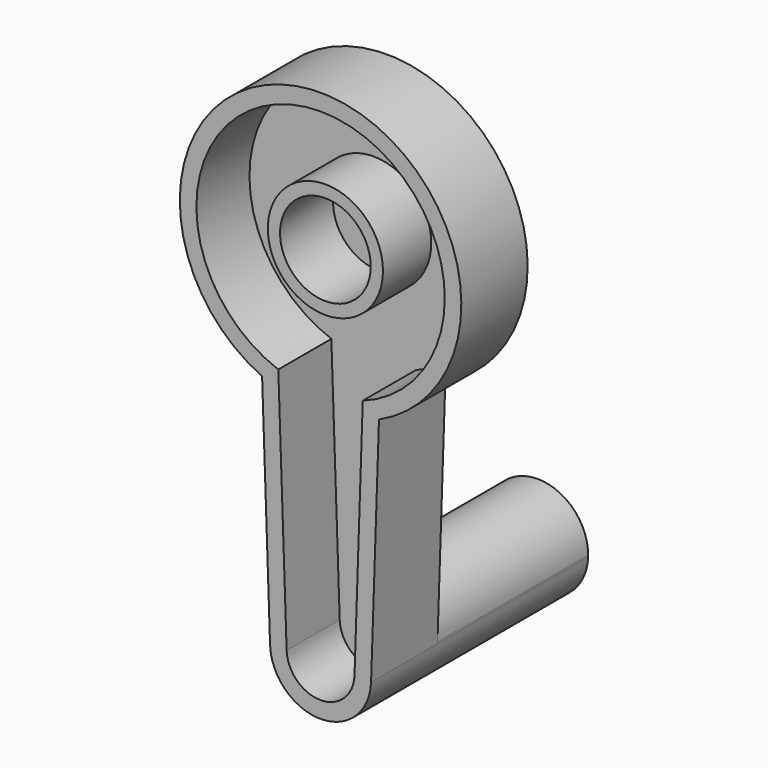
from build123d import *

# Parameters (mm, degrees)
F0_R     = 5.0192291216
F1_DEPTH = 11
F2_T     = -2.2
F3_R     = 7.6408252188
F4_DEPTH = 8
F5_R     = 6.0170563026
F6_DEPTH = 8.8
F7_DEPTH = 25


# Not quite as in the source:
# - a feature names something its author has since deleted; it is built from what else it names


with BuildPart() as f1:
    # F0 (on Front) → F1 (new body)
    with BuildSketch(Plane.XZ):
        with BuildLine():
            Line((6.7017039213, -13.6836004417), (7.7492278625, 17.3350542571))
            ThreePointArc((7.7492278625, 17.3350542571), (0.0056670875, 53.0044082442), (-7.7595389242, 17.3397601606))
            Line((-7.7595389242, 17.3397601606), (-6.7016295892, -13.6857909072))
            ThreePointArc((-6.7016295892, -13.6857909072), (-0.1142726876, -6.7527281229), (6.7055243621, -13.457278721))
            ThreePointArc((6.7055243621, -13.457278721), (6.7045691839, -13.570455703), (6.7017039213, -13.6836004417))
        make_face()
        with Locations((0, 34.3279652297)):
            Circle(F0_R, mode=Mode.SUBTRACT)
        with BuildLine():
            ThreePointArc((8.3308181793, 34.5567601339), (8.3292111279, 34.0466813329), (8.2964022532, 33.5376562417))
            Line((8.2964022532, 33.5376562417), (8.3308181793, 34.5567601339))
        make_face(mode=Mode.SUBTRACT)
        with BuildLine():
            ThreePointArc((-6.7016295892, -13.6857909072), (0.0010958632, -20.1628029936), (6.7017039213, -13.6836004417))
            ThreePointArc((6.7017039213, -13.6836004417), (6.7045691839, -13.570455703), (6.7055243621, -13.457278721))
            ThreePointArc((6.7055243621, -13.457278721), (-0.1142726876, -6.7527281229), (-6.7016295892, -13.6857909072))
        make_face()
        with BuildLine():
            Line((8.3308181793, 34.5567601339), (8.2964022532, 33.5376562417))
            ThreePointArc((8.2964022532, 33.5376562417), (8.3292111279, 34.0466813329), (8.3308181793, 34.5567601339))
        make_face()
        with Locations((0, 34.3279652297)):
            Circle(F0_R)
    extrude(amount=F1_DEPTH)

    # F2
    f2_openings = [f1.faces().sort_by_distance(p)[0] for p in [
        (-0.000731, -11, 23.334865),
    ]]
    offset(amount=F2_T, openings=f2_openings, kind=Kind.INTERSECTION)

    # F3 (on face) → F4 (join)
    with BuildSketch(Plane.XZ.offset(2.2)):
        with Locations((0, 34.3279652297)):
            Circle(F3_R)
    extrude(amount=F4_DEPTH)

    # F5 (on face) → F6 (cut)
    with BuildSketch(Plane.XZ.offset(10.2)):
        with Locations((0, 34.328058362)):
            Circle(F5_R)
    extrude(amount=-F6_DEPTH, mode=Mode.SUBTRACT)

    # F0 (on Front) → F7 (join)
    with BuildSketch(Plane.XZ):
        with BuildLine():
            ThreePointArc((-6.7016295892, -13.6857909072), (0.0010958632, -20.1628029936), (6.7017039213, -13.6836004417))
            ThreePointArc((6.7017039213, -13.6836004417), (6.7045691839, -13.570455703), (6.7055243621, -13.457278721))
            ThreePointArc((6.7055243621, -13.457278721), (-0.1142726876, -6.7527281229), (-6.7016295892, -13.6857909072))
        make_face()
    extrude(amount=-F7_DEPTH)


solid = f1.part
